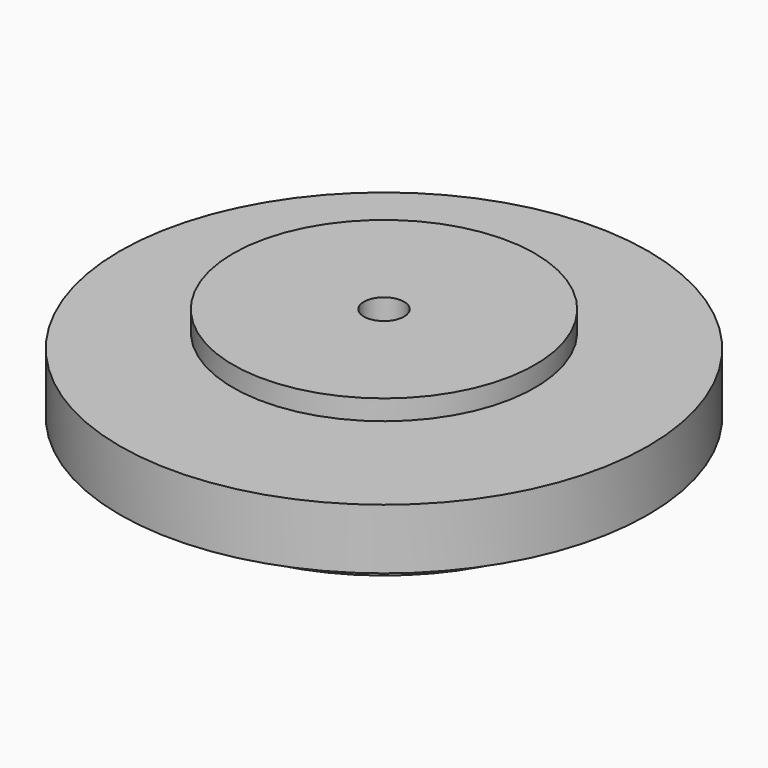
from build123d import *

# Parameters (mm, degrees)
F0_W            = 15
F0_H            = 6
F2_W            = 1.1
F2_H            = 7.7078238585
F3_DEPTH        = 83
F3_COPIES_COUNT = 3


# Not quite as in the source:
# - an extrude ends at something that could not be found from the text; its depth is read off the source's solid
# - a pattern or mirror of a feature is missing from the dataset's text; its kind, count and spacing are read off the source's solid


with BuildPart() as f1:
    # F0 (on Front) → F1 (revolve)
    with BuildSketch(Plane.XZ):
        Polygon((-2, -12.9), (-2, 0), (-15, 0), (-15, -2), (-5.8, -2), (-5.8, -2.8), (-3.7, -2.8), (-3.7, -12.2242640687), (-4.2, -12.7242640687), (-4.2, -12.9819470106), (-2, -14.0078238585), align=None)
    revolve(axis=Axis((0, 0, -0.0521782535), (0, 0, -1)))

    # F2 (on Right) → F3 (cut, through all)
    with BuildSketch(Plane.YZ):
        with Locations((0, -10.1539119293)):
            Rectangle(F2_W, F2_H)
    f3 = extrude(amount=F3_DEPTH, mode=Mode.SUBTRACT)

    # F3_copies: F3 ×3 about axis
    f3_copies_axis = Axis((0, 0, 0), (0, 0, 1))
    for i in range(1, F3_COPIES_COUNT):
        add(f3.rotate(f3_copies_axis, i * 360 / F3_COPIES_COUNT), mode=Mode.SUBTRACT)


with BuildPart() as f1b:
    # F0 (on Front) → F1, piece 2 (revolve)
    with BuildSketch(Plane.XZ):
        Polygon((-4.8, -12.9), (-4, -12.1), (-4, -10.1), (-4.8, -10.1), (-5.8, -10.1), (-5.8, -10.9), (-20, -10.9), (-20, -12.9), align=None)
    revolve(axis=Axis((0, 0, -0.0521782535), (0, 0, -1)))


with BuildPart() as f1c:
    # F0 (on Front) → F1, piece 3 (revolve)
    with BuildSketch(Plane.XZ):
        with Locations((-18.75, -6.45)):
            Rectangle(F0_W, F0_H)
    revolve(axis=Axis((0, 0, -0.0521782535), (0, 0, -1)))


solid = Compound([f1.part, f1b.part, f1c.part])
